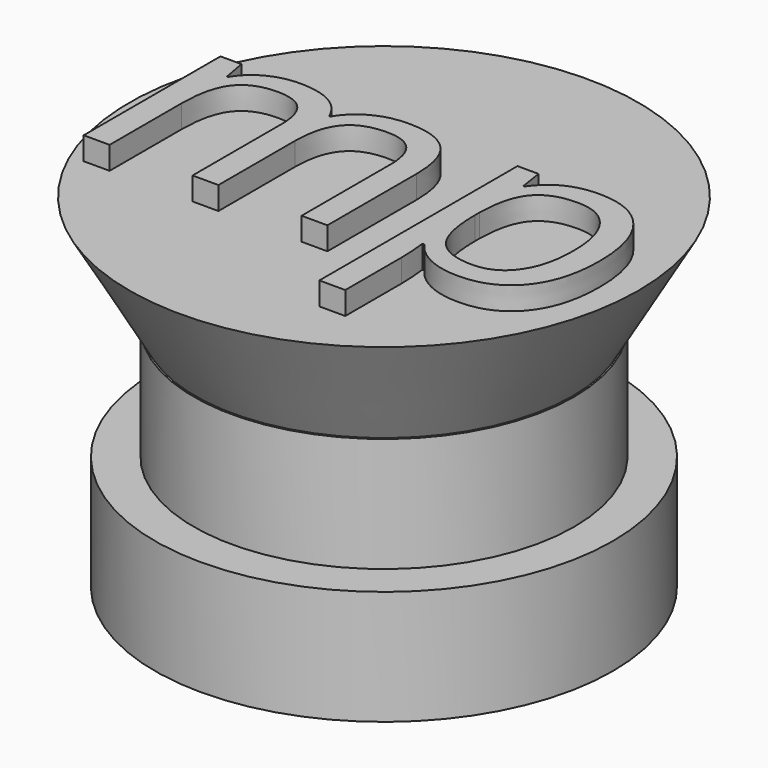
from build123d import *

# Parameters (mm, degrees)
F0_R         = 12.7
F1_DEPTH     = 6.35
F2_R         = 10.5545921867
F3_DEPTH     = 6.35
F4_R         = 10.4576710627
F4_R_2       = 10.2932855679
F5_DEPTH     = 6.35
F5_TAPER     = -30
F7_TEXT_SIZE = 17.7196369937
F8_DEPTH     = 1.27


# Not quite as in the source:
# - Text() gives the source's letters only with a copy of the font that has no kerning and outlines rounded to 1/6400 em; it was checked with that copy


with BuildPart() as f1:
    # F0 (on Top) → F1 (new body)
    with BuildSketch(Plane.XY):
        Circle(F0_R)
    extrude(amount=F1_DEPTH)

    # F2 (on face) → F3 (join)
    with BuildSketch(Plane.XY.offset(6.35)):
        Circle(F2_R)
    extrude(amount=F3_DEPTH)

    # F4 (on face) → F5 (join)
    with BuildSketch(Plane.XY.offset(12.7)):
        Circle(F4_R)
        Circle(F4_R_2, mode=Mode.SUBTRACT)
        Circle(F4_R_2)
    extrude(amount=F5_DEPTH, taper=F5_TAPER)

    # F7 (on face) → F8 (join)
    with BuildSketch(Plane.XY.offset(19.05)):
        with Locations((-13.7520995231, -5.5383248713)):
            Text('mp', F7_TEXT_SIZE, font='Open Sans', text_align=(TextAlign.LEFT, TextAlign.BOTTOM))
    extrude(amount=F8_DEPTH)


solid = f1.part
